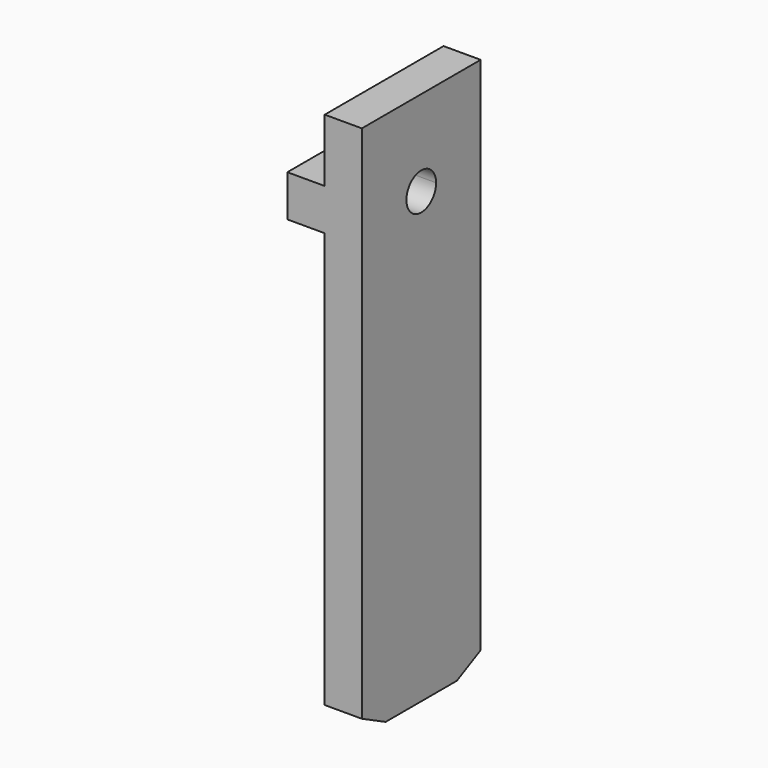
from build123d import *

# Parameters (mm, degrees)
F1_DEPTH = 25.4
F3_W     = 9.144
F3_H     = 7.112
F4_DEPTH = 6.3936169982
F5_DEPTH = 6.35
F6_SIZE2 = 2.54
F6_SIZE  = 5.08


with BuildPart() as f1:
    # F0 (on Front) → F1 (new body)
    with BuildSketch(Plane.XZ):
        Polygon((82.1067863703, 44.9580137503), (75.7567863703, 44.9580137503), (75.7567863703, 34.2138137503), (69.3631693721, 34.2138137503), (69.3631693721, 27.1018137503), (75.7567863703, 27.1018137503), (75.7567863703, -46.4819862497), (82.1067863703, -46.4819862497), align=None)
    extrude(amount=F1_DEPTH)

    # F3 (on face) → F4 (cut, through all)
    with BuildSketch(Plane(origin=(69.3631693721, 0, 0), x_dir=(0, -1, 0), z_dir=(-1, 0, 0))):
        with Locations((12.7, 30.6578137503)):
            Rectangle(F3_W, F3_H)
    extrude(amount=-F4_DEPTH, mode=Mode.SUBTRACT)

    # F2 (on face) → F5 (cut, through all)
    with BuildSketch(Plane.YZ.offset(82.1067863703)):
        with BuildLine():
            ThreePointArc((-9.525, 30.3022137503), (-10.4549359697, 32.5472777806), (-12.7, 33.4772137503))
            ThreePointArc((-12.7, 33.4772137503), (-14.9450640303, 28.05714972), (-9.525, 30.3022137503))
        make_face()
    extrude(amount=-F5_DEPTH, mode=Mode.SUBTRACT)

    # F6
    f6_edges = [f1.edges().sort_by_distance(p)[0] for p in [
        (78.931786, -25.4, -46.481986),
        (78.931786, 0, -46.481986),
    ]]
    f6_side = f1.faces().sort_by_distance((78.931786, -12.7, -46.481986))[0]
    chamfer(f6_edges, length=F6_SIZE, length2=F6_SIZE2, reference=f6_side)


solid = f1.part
